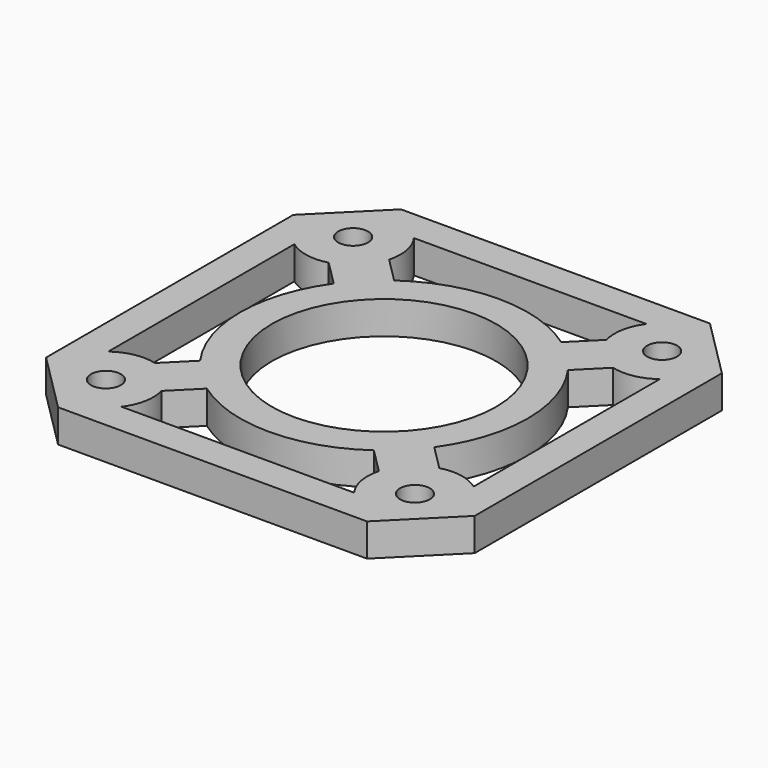
from build123d import *

# Parameters (mm, degrees)
F0_W            = 43.0059846
F0_H            = 43.0059846
F0_R            = 1.5
F0_R_2          = 11.2530001
F1_DEPTH        = 3.29057
F2_SIZE         = 6.0030106
F4_DEPTH        = 3.29057
F4_COPIES_COUNT = 4


# Not quite as in the source:
# - a pattern or mirror of a feature is missing from the dataset's text; its kind, count and spacing are read off the source's solid


with BuildPart() as f1:
    # F0 (on Top) → F1 (new body)
    with BuildSketch(Plane.XY):
        with Locations((21.5029923, 21.5029923)):
            Rectangle(F0_W, F0_H)
        with Locations((6.0029979, 6.0029979)):
            Circle(F0_R, mode=Mode.SUBTRACT)
        with Locations((21.5029923, 21.5029923)):
            Circle(F0_R_2, mode=Mode.SUBTRACT)
        with Locations((37.0029867, 6.0029979)):
            Circle(F0_R, mode=Mode.SUBTRACT)
        with Locations((6.0029979, 37.0029867)):
            Circle(F0_R, mode=Mode.SUBTRACT)
        with Locations((37.0029867, 37.0029867)):
            Circle(F0_R, mode=Mode.SUBTRACT)
    extrude(amount=F1_DEPTH)

    # F2
    f2_edges = [f1.edges().sort_by_distance(p)[0] for p in [
        (0, 0, 1.645285),
        (0, 43.005985, 1.645285),
        (43.005985, 0, 1.645285),
        (43.005985, 43.005985, 1.645285),
    ]]
    chamfer(f2_edges, length=F2_SIZE)

    # F3 (on face) → F4 (cut, through all)
    with BuildSketch(Plane.XY.offset(3.29057)):
        with BuildLine():
            ThreePointArc((7.2356236023, 32.4027649523), (5.1176370603, 32.3235056996), (3.175, 33.171037571))
            Line((3.175, 33.171037571), (3.175, 9.834947029))
            ThreePointArc((3.175, 9.834947029), (5.1176370603, 10.6824789004), (7.2356236023, 10.6032196477))
            Line((7.2356236023, 10.6032196477), (9.7569670059, 13.1245630513))
            ThreePointArc((9.7569670059, 13.1245630513), (7.0749922, 21.5029923), (9.7569670059, 29.8814215487))
            Line((9.7569670059, 29.8814215487), (7.2356236023, 32.4027649523))
        make_face()
    f4 = extrude(amount=-F4_DEPTH, mode=Mode.SUBTRACT)

    # F4_copies: F4 ×4 about axis
    f4_copies_axis = Axis((21.502992, 21.502992, 0), (0, 0, 1))
    for i in range(1, F4_COPIES_COUNT):
        add(f4.rotate(f4_copies_axis, i * 360 / F4_COPIES_COUNT), mode=Mode.SUBTRACT)


solid = f1.part
